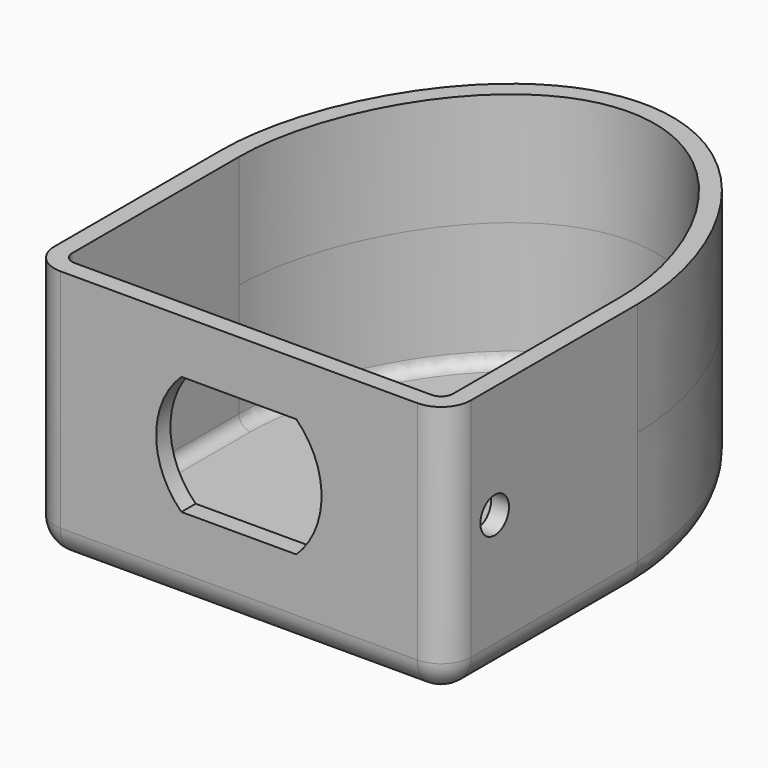
from build123d import *

# Parameters (mm, degrees)
F1_DEPTH  = 24
F4_R      = 5
F5_W      = 91.2617743015
F5_H      = 146.8465328217
F6_DEPTH  = 5
F7_T      = -3
F9_W      = 24
F9_H      = 37.5
F10_DEPTH = 2
F11_DEPTH = 3
F13_R     = 3
F15_DEPTH = 3
F14_R     = 3
F16_DEPTH = 3


with BuildPart() as f1:
    # F0 (on Top) → F1 (new body, symmetric)
    with BuildSketch(Plane.XY):
        with BuildLine():
            Line((-35, -1.2857098173), (-35, -41.2857098173))
            Line((-35, -41.2857098173), (35, -41.2857098173))
            Line((35, -41.2857098173), (35, -1.2857098173))
            add(Edge.make_bspline(
                [(0, 43.7142857143), (20.1986748725, 43.7142857143), (35, 18.7647750933), (35, -1.2857098173)],
                knots=[0, 0, 0, 0, 57.0087677278, 57.0087677278, 57.0087677278, 57.0087677278], degree=3))
            add(Edge.make_bspline(
                [(0, 43.7142857143), (-20.1986748725, 43.7142857143), (-35, 18.7647750933), (-35, -1.2857098173)],
                knots=[0, 0, 0, 0, 57.0087677278, 57.0087677278, 57.0087677278, 57.0087677278], degree=3))
        make_face()
    extrude(amount=F1_DEPTH, both=True)

    # F4
    f4_edges = [f1.edges().sort_by_distance(p)[0] for p in [
        (-35, -21.28571, -24),
        (-25.571688, 28.021772, -24),
        (0, -41.28571, 24),
        (-35, -21.28571, 24),
        (-35, -41.28571, 0),
        (35, -41.28571, 0),
        (0, -41.28571, -24),
    ]]
    fillet(f4_edges, radius=F4_R)

    # F5 (on face) → F6 (cut)
    with BuildSketch(Plane.XY.offset(24)):
        Rectangle(F5_W, F5_H)
    extrude(amount=-F6_DEPTH, mode=Mode.SUBTRACT)

    # F7
    f7_openings = [f1.faces().sort_by_distance(p)[0] for p in [
        (0, -3.179771, 19),
    ]]
    offset(amount=F7_T, openings=f7_openings, kind=Kind.INTERSECTION)

    # F9 (on face) → F10 (cut)
    with BuildSketch(Plane(origin=(0, 0, -24), x_dir=(1, 0, 0), z_dir=(0, 0, -1))):
        Rectangle(F9_W, F9_H)
    extrude(amount=-F10_DEPTH, mode=Mode.SUBTRACT)

    # F8 (on face) → F11 (cut)
    with BuildSketch(Plane.XZ.offset(41.2857098173)):
        with BuildLine():
            Line((9.6545326143, 10), (0, 10))
            Line((0, 10), (0, 0))
            Line((0, 0), (0, -10))
            Line((0, -10), (9.6545326143, -10))
            ThreePointArc((9.6545326143, -10), (13.9, 0), (9.6545326143, 10))
        make_face()
        with BuildLine():
            Line((0, 10), (-9.6545326143, 10))
            ThreePointArc((-9.6545326143, 10), (-13.9, 0), (-9.6545326143, -10))
            Line((-9.6545326143, -10), (0, -10))
            Line((0, -10), (0, 0))
            Line((0, 0), (0, 10))
        make_face()
    extrude(amount=-F11_DEPTH, mode=Mode.SUBTRACT)

    # F13 (on face) → F15 (cut)
    with BuildSketch(Plane(origin=(-35, 0, 0), x_dir=(0, -1, 0), z_dir=(-1, 0, 0))):
        with Locations((31.2857098173, 0)):
            Circle(F13_R)
    extrude(amount=-F15_DEPTH, mode=Mode.SUBTRACT)

    # F14 (on face) → F16 (cut)
    with BuildSketch(Plane.YZ.offset(35)):
        with Locations((-31.2857098173, 0)):
            Circle(F14_R)
    extrude(amount=-F16_DEPTH, mode=Mode.SUBTRACT)


solid = f1.part
